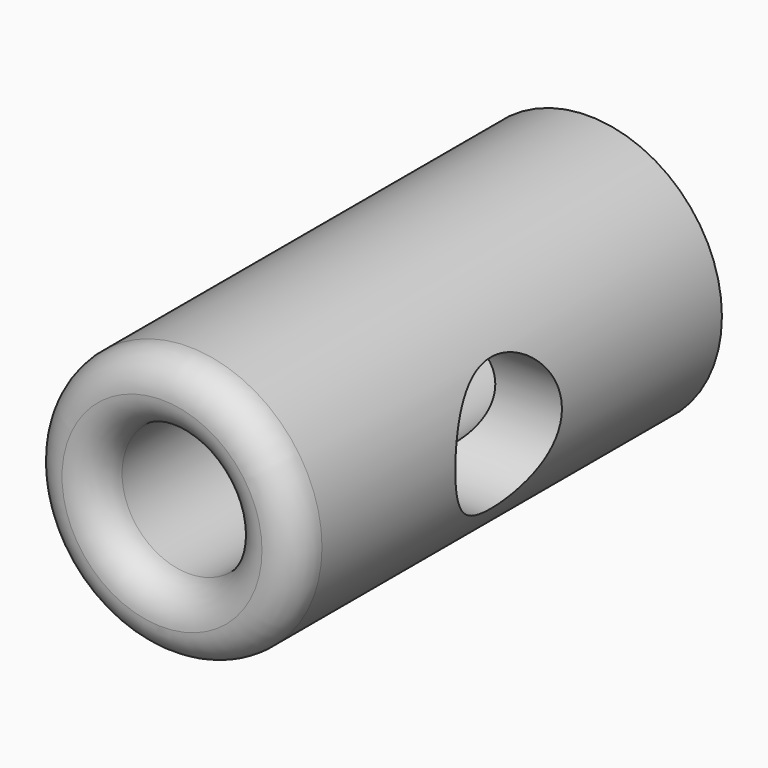
from build123d import *

# Parameters (mm, degrees)
F0_R     = 38.1
F0_R_2   = 19.05
F1_DEPTH = 76.2
F2_R     = 9.52499
F4_R     = 31.75
F4_R_2   = 25.4
F5_DEPTH = 3.175
F6_R     = 3.17499
F8_R     = 19.05
F9_DEPTH = 152.4


# Not quite as in the source:
# - a fillet or chamfer is up to 0.001 mm smaller than in the source, because OpenCascade refuses the exact size


with BuildPart() as f1:
    # F0 (on Front) → F1 (new body, symmetric)
    with BuildSketch(Plane.XZ):
        Circle(F0_R)
        Circle(F0_R_2, mode=Mode.SUBTRACT)
    extrude(amount=F1_DEPTH, both=True)

    # F2 (radius 9.525 in the source; OpenCascade refuses exactly that, so slightly less here)
    f2_edges = [f1.edges().sort_by_distance(p)[0] for p in [
        (-38.1, -76.2, 0),
        (-19.05, -76.2, 0),
    ]]
    fillet(f2_edges, radius=F2_R)

    # F4 (on offset) → F5 (cut)
    with BuildSketch(Plane(origin=(0, 76.2, 0), x_dir=(-1, 0, 0), z_dir=(0, 1, 0))):
        Circle(F4_R)
        Circle(F4_R_2, mode=Mode.SUBTRACT)
    extrude(amount=-F5_DEPTH, mode=Mode.SUBTRACT)

    # F6 (radius 3.175 in the source; OpenCascade refuses exactly that, so slightly less here)
    f6_edges = [f1.edges().sort_by_distance(p)[0] for p in [
        (31.75, 73.025, 0),
        (25.4, 73.025, 0),
    ]]
    fillet(f6_edges, radius=F6_R)

    # F8 (on offset) → F9 (cut)
    with BuildSketch(Plane.YZ.offset(76.2)):
        Circle(F8_R)
    extrude(amount=-F9_DEPTH, mode=Mode.SUBTRACT)


solid = f1.part
